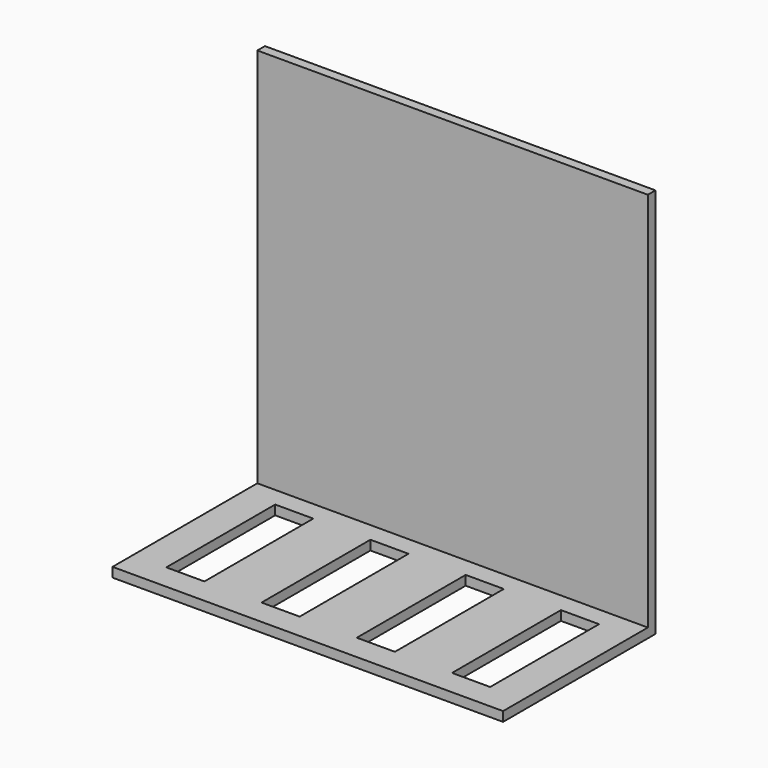
from build123d import *

# Parameters (mm, degrees)
F1_E0_W  = 40
F1_E0_H  = 82
F2_DEPTH = 2
F1_E1_W  = 82
F1_E1_H  = 82
F3_DEPTH = 2
F4_W     = 8
F4_H     = 28.5714303715
F5_DEPTH = 2.001


with BuildPart() as f2:
    # F1_E0 (on explicit) → F2 (new body)
    with BuildSketch(Plane(origin=(0, -48.5075005184, 0), x_dir=(0, 1, 0), z_dir=(0, 0, -1))):
        with Locations((20, 41)):
            Rectangle(F1_E0_W, F1_E0_H)
    extrude(amount=-F2_DEPTH)

    # F1_E1 (on explicit) → F3 (join)
    with BuildSketch(Plane.ZX.offset(-8.5075005184)):
        with Locations((41, 41)):
            Rectangle(F1_E1_W, F1_E1_H)
    extrude(amount=-F3_DEPTH)

    # F4 (on face) → F5 (cut, through all)
    with BuildSketch(Plane.XY.offset(2)):
        with Locations((71, -28.857444413)):
            Rectangle(F4_W, F4_H)
        with Locations((51, -28.857444413)):
            Rectangle(F4_W, F4_H)
        with Locations((31, -28.857444413)):
            Rectangle(F4_W, F4_H)
        with Locations((11, -28.857444413)):
            Rectangle(F4_W, F4_H)
    extrude(amount=-F5_DEPTH, mode=Mode.SUBTRACT)


solid = f2.part
